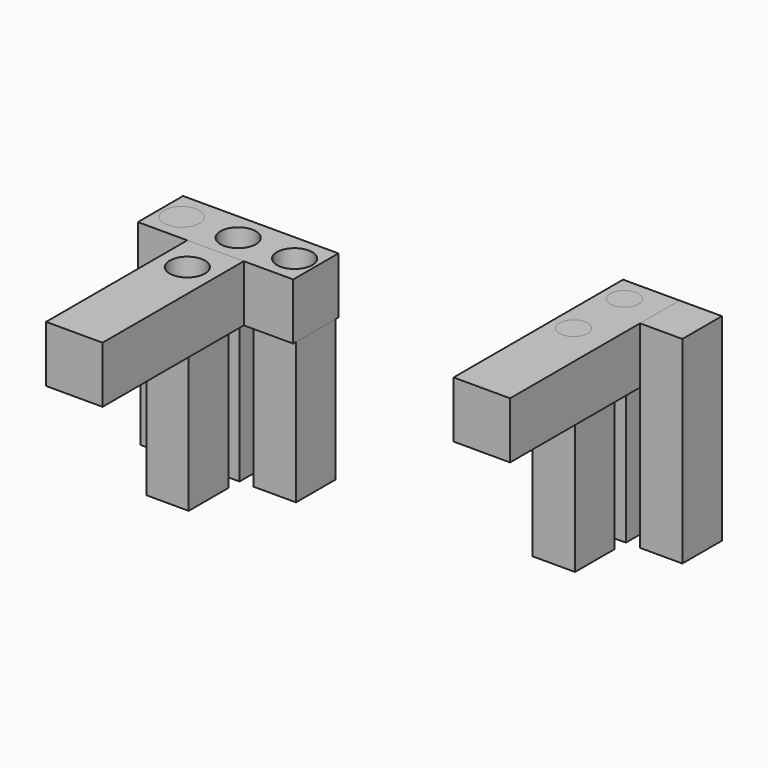
from build123d import *

# Parameters (mm, degrees)
F0_W      = 12
F0_H      = 14
F0_R      = 5
F1_DEPTH  = 16
F2_DEPTH  = 40
F0_W_2    = 16
F0_H_2    = 50
F3_DEPTH  = 16
F4_DEPTH  = 16
F0_R_2    = 4
F5_DEPTH  = 16
F6_DEPTH  = 16
F7_DEPTH  = 40
F8_DEPTH  = 40
F9_DEPTH  = 16
F10_DEPTH = 16
F11_DEPTH = 40


with BuildPart() as f1:
    # F0 (on Top) → F1 (new body)
    with BuildSketch(Plane.XY):
        Polygon((8, -8), (22, -8), (22, -7), (10, -7), (10, 7), (22, 7), (22, 8), (-22, 8), (-22, 7), (-10, 7), (-10, -7), (-22, -7), (-22, -8), (-8, -8), align=None)
        Rectangle(F0_W, F0_H, mode=Mode.SUBTRACT)
        with Locations((-16, 0)):
            Rectangle(F0_W, F0_H)
        with Locations((-16, 0)):
            Circle(F0_R, mode=Mode.SUBTRACT)
        Rectangle(F0_W, F0_H)
        Circle(F0_R, mode=Mode.SUBTRACT)
        with Locations((16, 0)):
            Rectangle(F0_W, F0_H)
        with Locations((16, 0)):
            Circle(F0_R, mode=Mode.SUBTRACT)
    extrude(amount=F1_DEPTH)


with BuildPart() as f2:
    # F0 (on Top) → F2 (new body)
    with BuildSketch(Plane.XY):
        with Locations((-16, 0)):
            Rectangle(F0_W, F0_H)
        with Locations((-16, 0)):
            Circle(F0_R, mode=Mode.SUBTRACT)
        with Locations((-16, 0)):
            Circle(F0_R)
    extrude(amount=-F2_DEPTH)

    # F0 (on Top) → F4 (join)
    with BuildSketch(Plane.XY):
        with Locations((-16, 0)):
            Circle(F0_R)
    extrude(amount=F4_DEPTH)


with BuildPart() as f2b:
    # F0 (on Top) → F2, piece 2 (new body)
    with BuildSketch(Plane.XY):
        Rectangle(F0_W, F0_H)
        Circle(F0_R, mode=Mode.SUBTRACT)
        Circle(F0_R)
    extrude(amount=-F2_DEPTH)


with BuildPart() as f2c:
    # F0 (on Top) → F2, piece 3 (new body)
    with BuildSketch(Plane.XY):
        with Locations((16, 0)):
            Rectangle(F0_W, F0_H)
        with Locations((16, 0)):
            Circle(F0_R, mode=Mode.SUBTRACT)
        with Locations((16, 0)):
            Circle(F0_R)
    extrude(amount=-F2_DEPTH)


with BuildPart() as f2d:
    # F0 (on Top) → F2, piece 4 (new body)
    with BuildSketch(Plane.XY):
        with Locations((0.0081723034, -18)):
            Rectangle(F0_W, F0_H)
        with Locations((0.0081723034, -18)):
            Circle(F0_R, mode=Mode.SUBTRACT)
        with Locations((0.0081723034, -18)):
            Circle(F0_R)
    extrude(amount=-F2_DEPTH)


with BuildPart() as f3:
    # F0 (on Top) → F3 (new body)
    with BuildSketch(Plane.XY):
        with Locations((0, -33)):
            Rectangle(F0_W_2, F0_H_2)
        with Locations((0.0081723034, -18)):
            Rectangle(F0_W, F0_H, mode=Mode.SUBTRACT)
        with Locations((0.0081723034, -18)):
            Rectangle(F0_W, F0_H)
        with Locations((0.0081723034, -18)):
            Circle(F0_R, mode=Mode.SUBTRACT)
    extrude(amount=F3_DEPTH)


with BuildPart() as f5:
    # F0 (on Top) → F5 (new body)
    with BuildSketch(Plane.XY):
        Polygon((79.0210366249, -22.486673668), (95.0210366249, -22.486673668), (95.0210366249, 23.513326332), (95.0210366249, 37.513326332), (91.0210366249, 37.513326332), (91.0210366249, 23.513326332), (79.0210366249, 23.513326332), (79.0210366249, 19.513326332), (91.0210366249, 19.513326332), (91.0210366249, 5.513326332), (79.0210366249, 5.513326332), align=None)
        with Locations((85.0210366249, 12.513326332)):
            Rectangle(F0_W, F0_H)
        with Locations((85.0210366249, 12.513326332)):
            Circle(F0_R_2, mode=Mode.SUBTRACT)
        with Locations((85.0210366249, 30.513326332)):
            Rectangle(F0_W, F0_H)
        with Locations((85.0210366249, 30.513326332)):
            Circle(F0_R_2, mode=Mode.SUBTRACT)
    extrude(amount=F5_DEPTH)


with BuildPart() as f6:
    # F0 (on Top) → F6 (new body)
    with BuildSketch(Plane.XY):
        with Locations((101.0210366249, 30.513326332)):
            Rectangle(F0_W, F0_H)
    extrude(amount=F6_DEPTH)

    # F0 (on Top) → F7 (join)
    with BuildSketch(Plane.XY):
        with Locations((101.0210366249, 30.513326332)):
            Rectangle(F0_W, F0_H)
    extrude(amount=-F7_DEPTH)


with BuildPart() as f8:
    # F0 (on Top) → F8 (new body)
    with BuildSketch(Plane.XY):
        with Locations((85.0210366249, 30.513326332)):
            Rectangle(F0_W, F0_H)
        with Locations((85.0210366249, 30.513326332)):
            Circle(F0_R_2, mode=Mode.SUBTRACT)
        with Locations((85.0210366249, 30.513326332)):
            Circle(F0_R_2)
    extrude(amount=-F8_DEPTH)

    # F0 (on Top) → F9 (join)
    with BuildSketch(Plane.XY):
        with Locations((85.0210366249, 30.513326332)):
            Circle(F0_R_2)
    extrude(amount=F9_DEPTH)


with BuildPart() as f10:
    # F0 (on Top) → F10 (new body)
    with BuildSketch(Plane.XY):
        with Locations((85.0210366249, 12.513326332)):
            Circle(F0_R_2)
    extrude(amount=F10_DEPTH)

    # F0 (on Top) → F11 (join)
    with BuildSketch(Plane.XY):
        with Locations((85.0210366249, 12.513326332)):
            Rectangle(F0_W, F0_H)
        with Locations((85.0210366249, 12.513326332)):
            Circle(F0_R_2, mode=Mode.SUBTRACT)
        with Locations((85.0210366249, 12.513326332)):
            Circle(F0_R_2)
    extrude(amount=-F11_DEPTH)


solid = Compound([f1.part, f2.part, f2b.part, f2c.part, f2d.part, f3.part, f5.part, f6.part, f8.part, f10.part])
